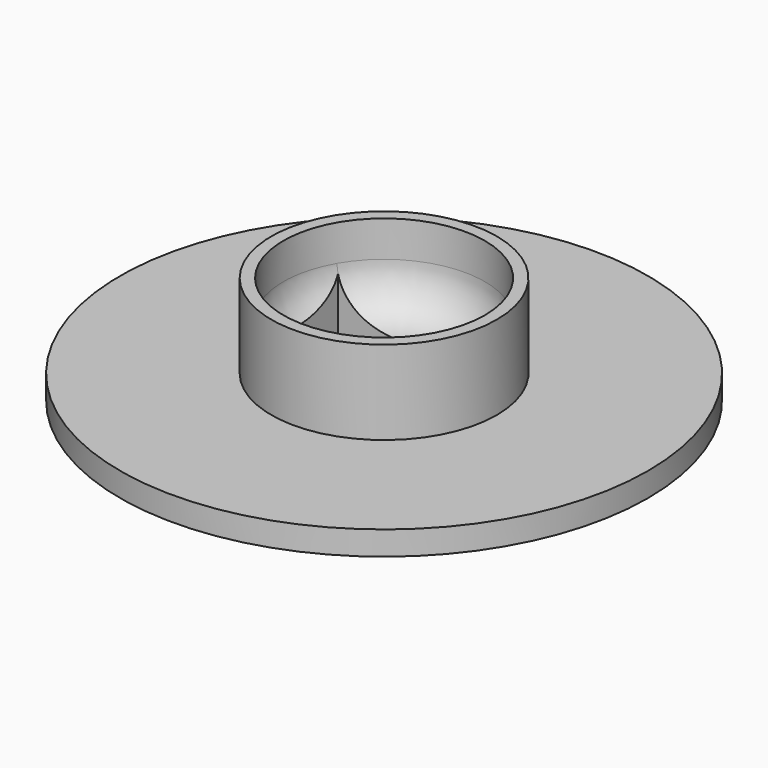
from build123d import *

# Parameters (mm, degrees)
F0_R     = 11
F0_W     = 7.2
F0_H     = 4.2
F1_DEPTH = 1
F2_R     = 4.7
F2_R_2   = 4.2
F3_DEPTH = 3.5


# Not quite as in the source:
# - a fillet or chamfer that OpenCascade refuses, or shapes differently, is made with other operations: its cross-section is extruded or revolved along the edge and cut away or added


with BuildPart() as f1:
    # F0 (on Top) → F1 (new body)
    with BuildSketch(Plane.XY):
        Circle(F0_R)
        Rectangle(F0_W, F0_H, mode=Mode.SUBTRACT)
    extrude(amount=F1_DEPTH)

    # F2 (on face) → F3 (join)
    with BuildSketch(Plane.XY.offset(1)):
        Circle(F2_R)
        Circle(F2_R_2, mode=Mode.SUBTRACT)
    extrude(amount=F3_DEPTH)

    # F4: fillet of radius 2 on 1 edges, made by hand


with BuildPart() as f4_tool2:
    # F4_s3 → F4_t4 (revolve)
    with BuildSketch(Plane.XZ):
        with BuildLine():
            ThreePointArc((2.2, 1), (3.6142135624, 1.5857864376), (4.2, 3))
            Line((4.2, 3), (4.2, 1))
            Line((4.2, 1), (2.2, 1))
        make_face()
    revolve(axis=Axis((0, 0, 1), (0, 0, 1)))

    split(bisect_by=Plane.YZ.offset(3.6), keep=Keep.TOP)


with BuildPart() as f1_1:
    add(f1.part)

    # F4_t1: union F4_tool2
    add(f4_tool2.part)


with BuildPart() as f4_tool7:
    # F4_s8 → F4_t9 (revolve)
    with BuildSketch(Plane.XZ):
        with BuildLine():
            ThreePointArc((2.2, 1), (3.6142135624, 1.5857864376), (4.2, 3))
            Line((4.2, 3), (4.2, 1))
            Line((4.2, 1), (2.2, 1))
        make_face()
    revolve(axis=Axis((0, 0, 1), (0, 0, 1)))

    split(bisect_by=Plane.XZ.offset(-2.1), keep=Keep.BOTTOM)


with BuildPart() as f1_2:
    add(f1_1.part)

    # F4_t6: union F4_tool7
    add(f4_tool7.part)


with BuildPart() as f4_tool12:
    # F4_s13 → F4_t14 (revolve)
    with BuildSketch(Plane.XZ):
        with BuildLine():
            ThreePointArc((2.2, 1), (3.6142135624, 1.5857864376), (4.2, 3))
            Line((4.2, 3), (4.2, 1))
            Line((4.2, 1), (2.2, 1))
        make_face()
    revolve(axis=Axis((0, 0, 1), (0, 0, 1)))

    split(bisect_by=Plane.XZ.offset(2.1), keep=Keep.TOP)


with BuildPart() as f1_3:
    add(f1_2.part)

    # F4_t11: union F4_tool12
    add(f4_tool12.part)


with BuildPart() as f4_tool17:
    # F4_s18 → F4_t19 (revolve)
    with BuildSketch(Plane.XZ):
        with BuildLine():
            ThreePointArc((2.2, 1), (3.6142135624, 1.5857864376), (4.2, 3))
            Line((4.2, 3), (4.2, 1))
            Line((4.2, 1), (2.2, 1))
        make_face()
    revolve(axis=Axis((0, 0, 1), (0, 0, 1)))

    split(bisect_by=Plane.YZ.offset(-3.6), keep=Keep.BOTTOM)


with BuildPart() as f1_4:
    add(f1_3.part)

    # F4_t16: union F4_tool17
    add(f4_tool17.part)


solid = f1_4.part
